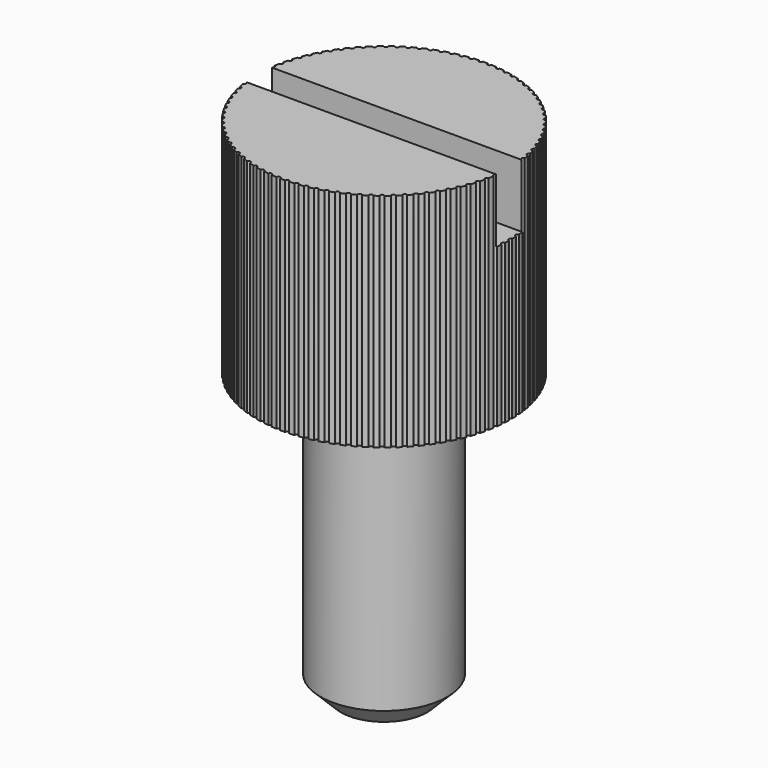
from build123d import *

# Parameters (mm, degrees)
F0_R     = 2
F1_DEPTH = 9
F2_R     = 4
F3_DEPTH = 7
F4_W     = 9
F4_H     = 1
F5_DEPTH = 2
F6_SIZE  = 0.635
F8_D     = 0.12


# Not quite as in the source:
# - a feature names something its author has since deleted; it is built from what else it names


with BuildPart() as f1:
    # F0 (on Top) → F1 (new body)
    with BuildSketch(Plane.XY):
        Circle(F0_R)
    extrude(amount=-F1_DEPTH)

    # F2 (on Top) → F3 (join)
    with BuildSketch(Plane.XY):
        Circle(F2_R)
    extrude(amount=F3_DEPTH)

    # F4 (on face) → F5 (cut)
    with BuildSketch(Plane.XY.offset(7)):
        Rectangle(F4_W, F4_H)
    extrude(amount=-F5_DEPTH, mode=Mode.SUBTRACT)

    # F6
    f6_edges = [f1.edges().sort_by_distance(p)[0] for p in [
        (-2, 0, -9),
    ]]
    chamfer(f6_edges, length=F6_SIZE)

    # F8 (through all)
    with Locations(Plane(origin=(0, 0, 0), x_dir=(1, 0, 0), z_dir=(0, 0, -1))):
        with Locations((4, 0), (-0.4181138531, 3.9780875815), (0.1395979868, 3.9975633081), (-2.2367716139, 3.3161502902), (-3.961072275, -0.5566924038), (2.6765224254, 2.9725793019), (2.8773592014, 2.7786334818), (3.0641777725, 2.5711504387), (3.2360679775, 2.3511410092), (-1.4984263737, 3.7087354183), (1.4984263737, 3.7087354183), (3.5317903714, 1.8778862511), (-3.8450467838, -1.1025494233), (0.4181138531, 3.9780875815), (1.2360679775, 3.8042260652), (0.9676875824, 3.8811829051), (-1.7534845872, 3.5951761852), (0.6945927107, 3.939231012), (-0.1395979868, 3.9975633081), (2.4626459013, 3.1520430144), (-3.9125904029, -0.8316467633), (1.7534845872, 3.5951761852), (2.2367716139, 3.3161502902), (2, 3.4641016151), (-1.2360679775, 3.8042260652), (-2, 3.4641016151), (3.3921923846, 2.1196770569), (3.6541818306, 1.6269465723), (3.7587704831, 1.3680805733), (3.8450467838, 1.1025494233), (3.9125904029, 0.8316467633), (3.961072275, 0.5566924038), (3.990256201, 0.279025895), (1.2360679775, -3.8042260652), (3.990256201, -0.279025895), (1.4984263737, -3.7087354183), (3.961072275, -0.5566924038), (-0.4181138531, -3.9780875815), (2.8773592014, -2.7786334818), (0.6945927107, -3.939231012), (2.2367716139, -3.3161502902), (3.2360679775, -2.3511410092), (2.6765224254, -2.9725793019), (0.4181138531, -3.9780875815), (3.3921923846, -2.1196770569), (-0.1395979868, -3.9975633081), (3.5317903714, -1.8778862511), (1.7534845872, -3.5951761852), (0.1395979868, -3.9975633081), (2.4626459013, -3.1520430144), (3.6541818306, -1.6269465723), (3.9125904029, -0.8316467633), (0.9676875824, -3.8811829051), (-0.9676875824, -3.8811829051), (3.0641777725, -2.5711504387), (2, -3.4641016151), (3.8450467838, -1.1025494233), (3.7587704831, -1.3680805733), (-2.6765224254, -2.9725793019), (-3.2360679775, -2.3511410092), (-2, -3.4641016151), (-3.3921923846, -2.1196770569), (-2.8773592014, -2.7786334818), (-3.7587704831, -1.3680805733), (-3.6541818306, -1.6269465723), (-2.4626459013, -3.1520430144), (-4, 0), (-3.5317903714, -1.8778862511), (-3.0641777725, -2.5711504387), (-3.990256201, -0.279025895), (-1.2360679775, -3.8042260652), (-1.4984263737, -3.7087354183), (-1.7534845872, -3.5951761852), (-2.2367716139, -3.3161502902), (-0.6945927107, -3.939231012), (-3.7587704831, 1.3680805733), (-3.990256201, 0.279025895), (-3.8450467838, 1.1025494233), (-0.6945927107, 3.939231012), (-3.0641777725, 2.5711504387), (-3.9125904029, 0.8316467633), (-0.9676875824, 3.8811829051), (-3.2360679775, 2.3511410092), (-3.6541818306, 1.6269465723), (-2.4626459013, 3.1520430144), (-3.961072275, 0.5566924038), (-3.5317903714, 1.8778862511), (-2.6765224254, 2.9725793019), (-3.3921923846, 2.1196770569), (-2.8773592014, 2.7786334818)):
            Hole(F8_D / 2)


solid = f1.part
